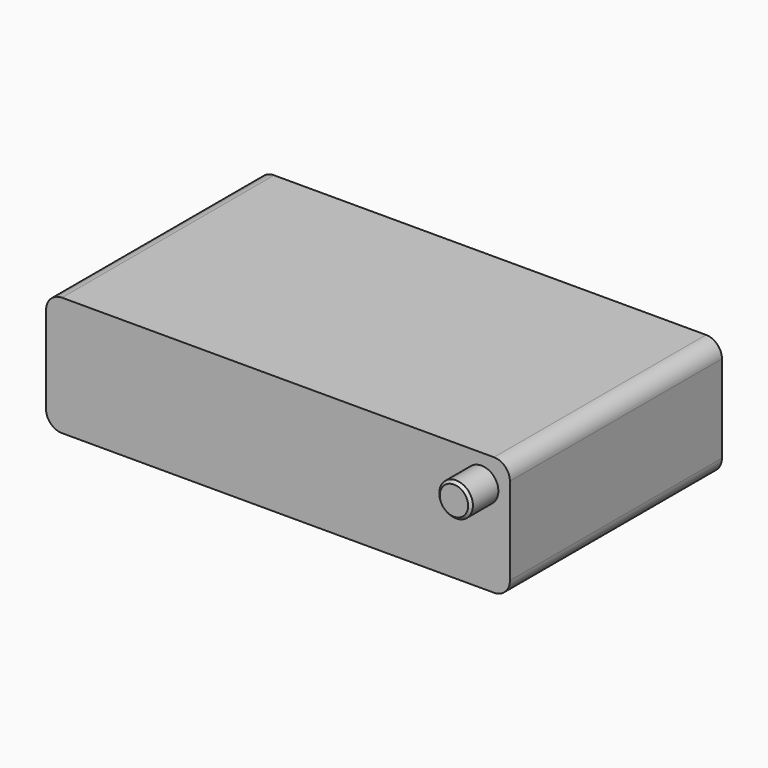
from build123d import *

# Parameters (mm, degrees)
F0_W     = 175
F0_H     = 100
F1_DEPTH = 45.0088
F2_R     = 6.35
F3_DEPTH = 13
F4_SIZE  = 1
F5_R     = 6
F6_W     = 19.05
F6_H     = 82.55
F7_DEPTH = 1.5875
F8_R     = 9.52499


# Not quite as in the source:
# - a fillet or chamfer is up to 0.001 mm smaller than in the source, because OpenCascade refuses the exact size
# - a length typed as a fraction of an inch, garbled in the dataset ("3 / 203.2 mm" for 3/8 in), is restored
# - a pattern or mirror of a feature is missing from the dataset's text; its kind, count and spacing are read off the source's solid


with BuildPart() as f1:
    # F0 (on Top) → F1 (new body)
    with BuildSketch(Plane.XY):
        Rectangle(F0_W, F0_H)
    extrude(amount=F1_DEPTH)

    # F2 (on face) → F3 (join)
    with BuildSketch(Plane.XZ.offset(50)):
        with Locations((76.7980482321, 34.3557204665)):
            Circle(F2_R)
    extrude(amount=F3_DEPTH)

    # F4
    f4_edges = [f1.edges().sort_by_distance(p)[0] for p in [
        (70.448048, -63, 34.35572),
    ]]
    chamfer(f4_edges, length=F4_SIZE)

    # F5
    f5_edges = [f1.edges().sort_by_distance(p)[0] for p in [
        (-87.5, 0, 45.0088),
        (87.5, 0, 45.0088),
        (87.5, 0, 0),
        (-87.5, 0, 0),
    ]]
    fillet(f5_edges, radius=F5_R)

    # F6 (on face) → F7 (join)
    with BuildSketch(Plane(origin=(0, 0, 0), x_dir=(1, 0, 0), z_dir=(0, 0, -1))):
        with Locations((-66.8625, 0)):
            Rectangle(F6_W, F6_H)
    f7 = extrude(amount=F7_DEPTH)

    # F7_copies: F7 across plane
    add(f7.mirror(Plane(origin=(0, 0, 0), x_dir=(0, 0, 1), z_dir=(1, 0, 0))))

    # F8 (radius 9.525 in the source; OpenCascade refuses exactly that, so slightly less here)
    f8_edges = [f1.edges().sort_by_distance(p)[0] for p in [
        (-76.3875, -41.275, -0.79375),
        (-57.3375, -41.275, -0.79375),
        (-76.3875, 41.275, -0.79375),
        (-57.3375, 41.275, -0.79375),
        (76.3875, -41.275, -0.79375),
        (76.3875, 41.275, -0.79375),
        (57.3375, 41.275, -0.79375),
        (57.3375, -41.275, -0.79375),
    ]]
    fillet(f8_edges, radius=F8_R)


solid = f1.part
